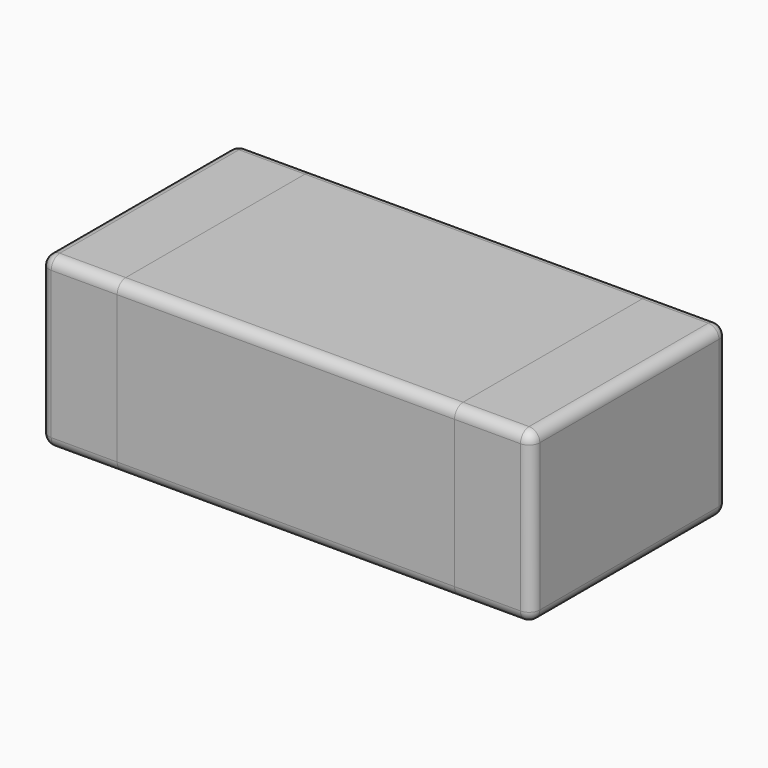
from build123d import *

# Parameters (mm, degrees)
F0_W           = 0.5
F0_H           = 1.6
F1_DEPTH       = 1.1
F0_W_2         = 2.2
F2_DEPTH       = 1.1
F3_R           = 0.07
F3_2_R         = 0.07
F4_T1_DEPTH    = 0.605
F4_S5_W        = 0.07
F4_S5_H        = 0.07
F4_T6_DEPTH    = 0.07
F4_S11_W       = 0.07
F4_S11_H       = 0.07
F4_T12_DEPTH   = 0.07
F4_S17_W       = 0.07
F4_S17_H       = 0.07
F4_T18_DEPTH   = 0.07
F4_S23_W       = 0.07
F4_S23_H       = 0.07
F4_T24_DEPTH   = 0.07
F4_2_F1_R      = 0.07
F4_2_F2_R      = 0.07
F4_2_F3_R      = 0.07
F4_2_F4_R      = 0.07
F4_3_T1_DEPTH  = 0.605
F4_3_S5_W      = 0.07
F4_3_S5_H      = 0.07
F4_3_T6_DEPTH  = 0.07
F4_3_S11_W     = 0.07
F4_3_S11_H     = 0.07
F4_3_T12_DEPTH = 0.07
F4_3_S17_W     = 0.07
F4_3_S17_H     = 0.07
F4_3_T18_DEPTH = 0.07
F4_3_S23_W     = 0.07
F4_3_S23_H     = 0.07
F4_3_T24_DEPTH = 0.07


# Not quite as in the source:
# - a fillet or chamfer that OpenCascade refuses, or shapes differently, is made with other operations: its cross-section is extruded or revolved along the edge and cut away or added


with BuildPart() as f1:
    # F0 (on Top) → F1 (new body)
    with BuildSketch(Plane.XY):
        with Locations((-1.35, 0)):
            Rectangle(F0_W, F0_H)
    extrude(amount=F1_DEPTH)

    # F3#2
    f3_2_edges = [f1.edges().sort_by_distance(p)[0] for p in [
        (-1.6, 0.8, 0.55),
        (-1.6, -0.8, 0.55),
        (-1.6, 0, 0),
        (-1.6, 0, 1.1),
    ]]
    fillet(f3_2_edges, radius=F3_2_R)

    # F4#3: fillet of radius 0.07 on 4 edges, made by hand

    # F4_3_s2 → F4_3_t1 (cut)
    with BuildSketch(Plane.YZ.offset(-1.53)):
        with BuildLine():
            ThreePointArc((0.73, 1.1), (0.7794974747, 1.0794974747), (0.8, 1.03))
            Line((0.8, 1.03), (0.8, 1.1))
            Line((0.8, 1.1), (0.73, 1.1))
        make_face()
        with BuildLine():
            ThreePointArc((0.73, 0), (0.7794974747, 0.0205025253), (0.8, 0.07))
            Line((0.8, 0.07), (0.8, 0))
            Line((0.8, 0), (0.73, 0))
        make_face()
        with BuildLine():
            ThreePointArc((-0.8, 1.03), (-0.7794974747, 1.0794974747), (-0.73, 1.1))
            Line((-0.73, 1.1), (-0.8, 1.1))
            Line((-0.8, 1.1), (-0.8, 1.03))
        make_face()
        with BuildLine():
            ThreePointArc((-0.8, 0.07), (-0.7794974747, 0.0205025253), (-0.73, 0))
            Line((-0.73, 0), (-0.8, 0))
            Line((-0.8, 0), (-0.8, 0.07))
        make_face()
    extrude(amount=F4_3_T1_DEPTH, mode=Mode.SUBTRACT)


with BuildPart() as f1b:
    # F0 (on Top) → F1, piece 2 (new body)
    with BuildSketch(Plane.XY):
        with Locations((1.35, 0)):
            Rectangle(F0_W, F0_H)
    extrude(amount=F1_DEPTH)

    # F3
    f3_edges = [f1b.edges().sort_by_distance(p)[0] for p in [
        (1.6, -0.8, 0.55),
        (1.6, 0.8, 0.55),
        (1.6, 0, 0),
        (1.6, 0, 1.1),
    ]]
    fillet(f3_edges, radius=F3_R)

    # F4: fillet of radius 0.07 on 4 edges, made by hand

    # F4_s2 → F4_t1 (cut)
    with BuildSketch(Plane.YZ.offset(0.925)):
        with BuildLine():
            ThreePointArc((0.73, 1.1), (0.7794974747, 1.0794974747), (0.8, 1.03))
            Line((0.8, 1.03), (0.8, 1.1))
            Line((0.8, 1.1), (0.73, 1.1))
        make_face()
        with BuildLine():
            ThreePointArc((0.73, 0), (0.7794974747, 0.0205025253), (0.8, 0.07))
            Line((0.8, 0.07), (0.8, 0))
            Line((0.8, 0), (0.73, 0))
        make_face()
        with BuildLine():
            ThreePointArc((-0.8, 1.03), (-0.7794974747, 1.0794974747), (-0.73, 1.1))
            Line((-0.73, 1.1), (-0.8, 1.1))
            Line((-0.8, 1.1), (-0.8, 1.03))
        make_face()
        with BuildLine():
            ThreePointArc((-0.8, 0.07), (-0.7794974747, 0.0205025253), (-0.73, 0))
            Line((-0.73, 0), (-0.8, 0))
            Line((-0.8, 0), (-0.8, 0.07))
        make_face()
    extrude(amount=F4_T1_DEPTH, mode=Mode.SUBTRACT)


with BuildPart() as f2:
    # F0 (on Top) → F2 (new body)
    with BuildSketch(Plane.XY):
        Rectangle(F0_W_2, F0_H)
    extrude(amount=F2_DEPTH)

    # F4#2: fillet of radius 0.07 on 4 edges, made by hand

    # F4_2_f1
    f4_2_f1_edges = [f2.edges().sort_by_distance(p)[0] for p in [
        (0, -0.8, 0),
    ]]
    fillet(f4_2_f1_edges, radius=F4_2_F1_R)

    # F4_2_f2
    f4_2_f2_edges = [f2.edges().sort_by_distance(p)[0] for p in [
        (0, -0.8, 1.1),
    ]]
    fillet(f4_2_f2_edges, radius=F4_2_F2_R)

    # F4_2_f3
    f4_2_f3_edges = [f2.edges().sort_by_distance(p)[0] for p in [
        (0, 0.8, 0),
    ]]
    fillet(f4_2_f3_edges, radius=F4_2_F3_R)

    # F4_2_f4
    f4_2_f4_edges = [f2.edges().sort_by_distance(p)[0] for p in [
        (0, 0.8, 1.1),
    ]]
    fillet(f4_2_f4_edges, radius=F4_2_F4_R)


with BuildPart() as f4_tool4:
    # F4_s5 → F4_t6 (new body)
    with BuildSketch(Plane.XZ.offset(0.73)):
        with Locations((1.565, 0.035)):
            Rectangle(F4_S5_W, F4_S5_H)
    extrude(amount=F4_T6_DEPTH)

    # F4_s7 → F4_t8 (revolve, cut)
    with BuildSketch(Plane(origin=(1.53, -0.73, 0.07), x_dir=(-0.7071067812, 0, 0.7071067812), z_dir=(0.7071067812, 0, 0.7071067812))):
        with BuildLine():
            ThreePointArc((0, -0.07), (0.07, 0), (0, 0.07))
            Line((0, 0.07), (0, -0.07))
        make_face()
    revolve(axis=Axis((1.53, -0.73, 0.07), (0, -1, 0)), mode=Mode.SUBTRACT)


with BuildPart() as f1b_1:
    add(f1b.part)

    # F4_t3: cut F4_tool4
    add(f4_tool4.part, mode=Mode.SUBTRACT)


with BuildPart() as f4_tool10:
    # F4_s11 → F4_t12 (new body)
    with BuildSketch(Plane.XZ.offset(0.73)):
        with Locations((1.565, 1.065)):
            Rectangle(F4_S11_W, F4_S11_H)
    extrude(amount=F4_T12_DEPTH)

    # F4_s13 → F4_t14 (revolve, cut)
    with BuildSketch(Plane(origin=(1.53, -0.73, 1.03), x_dir=(-0.7071067812, 0, -0.7071067812), z_dir=(-0.7071067812, 0, 0.7071067812))):
        with BuildLine():
            ThreePointArc((0, -0.07), (0.07, 0), (0, 0.07))
            Line((0, 0.07), (0, -0.07))
        make_face()
    revolve(axis=Axis((1.53, -0.73, 1.03), (0, -1, 0)), mode=Mode.SUBTRACT)


with BuildPart() as f1b_2:
    add(f1b_1.part)

    # F4_t9: cut F4_tool10
    add(f4_tool10.part, mode=Mode.SUBTRACT)


with BuildPart() as f4_tool16:
    # F4_s17 → F4_t18 (new body)
    with BuildSketch(Plane.XY.offset(0.07)):
        with Locations((1.565, 0.765)):
            Rectangle(F4_S17_W, F4_S17_H)
    extrude(amount=-F4_T18_DEPTH)

    # F4_s19 → F4_t20 (revolve, cut)
    with BuildSketch(Plane(origin=(1.53, 0.73, 0.07), x_dir=(-0.7071067812, -0.7071067812, 0), z_dir=(0.7071067812, -0.7071067812, 0))):
        with BuildLine():
            ThreePointArc((0, -0.07), (0.07, 0), (0, 0.07))
            Line((0, 0.07), (0, -0.07))
        make_face()
    revolve(axis=Axis((1.53, 0.73, 0.07), (0, 0, -1)), mode=Mode.SUBTRACT)


with BuildPart() as f1b_3:
    add(f1b_2.part)

    # F4_t15: cut F4_tool16
    add(f4_tool16.part, mode=Mode.SUBTRACT)


with BuildPart() as f4_tool22:
    # F4_s23 → F4_t24 (new body)
    with BuildSketch(Plane.XY.offset(1.03)):
        with Locations((1.565, 0.765)):
            Rectangle(F4_S23_W, F4_S23_H)
    extrude(amount=F4_T24_DEPTH)

    # F4_s25 → F4_t26 (revolve, cut)
    with BuildSketch(Plane(origin=(1.53, 0.73, 1.03), x_dir=(-0.7071067812, -0.7071067812, 0), z_dir=(-0.7071067812, 0.7071067812, 0))):
        with BuildLine():
            ThreePointArc((0, -0.07), (0.07, 0), (0, 0.07))
            Line((0, 0.07), (0, -0.07))
        make_face()
    revolve(axis=Axis((1.53, 0.73, 1.03), (0, 0, 1)), mode=Mode.SUBTRACT)


with BuildPart() as f1b_4:
    add(f1b_3.part)

    # F4_t21: cut F4_tool22
    add(f4_tool22.part, mode=Mode.SUBTRACT)


with BuildPart() as f4_3_tool4:
    # F4_3_s5 → F4_3_t6 (new body)
    with BuildSketch(Plane.XZ.offset(0.73)):
        with Locations((-1.565, 0.035)):
            Rectangle(F4_3_S5_W, F4_3_S5_H)
    extrude(amount=F4_3_T6_DEPTH)

    # F4_3_s7 → F4_3_t8 (revolve, cut)
    with BuildSketch(Plane(origin=(-1.53, -0.73, 0.07), x_dir=(0.7071067812, 0, 0.7071067812), z_dir=(0.7071067812, 0, -0.7071067812))):
        with BuildLine():
            ThreePointArc((0, -0.07), (0.07, 0), (0, 0.07))
            Line((0, 0.07), (0, -0.07))
        make_face()
    revolve(axis=Axis((-1.53, -0.73, 0.07), (0, -1, 0)), mode=Mode.SUBTRACT)


with BuildPart() as f1_1:
    add(f1.part)

    # F4_3_t3: cut F4_3_tool4
    add(f4_3_tool4.part, mode=Mode.SUBTRACT)


with BuildPart() as f4_3_tool10:
    # F4_3_s11 → F4_3_t12 (new body)
    with BuildSketch(Plane.XZ.offset(0.73)):
        with Locations((-1.565, 1.065)):
            Rectangle(F4_3_S11_W, F4_3_S11_H)
    extrude(amount=F4_3_T12_DEPTH)

    # F4_3_s13 → F4_3_t14 (revolve, cut)
    with BuildSketch(Plane(origin=(-1.53, -0.73, 1.03), x_dir=(0.7071067812, 0, -0.7071067812), z_dir=(-0.7071067812, 0, -0.7071067812))):
        with BuildLine():
            ThreePointArc((0, -0.07), (0.07, 0), (0, 0.07))
            Line((0, 0.07), (0, -0.07))
        make_face()
    revolve(axis=Axis((-1.53, -0.73, 1.03), (0, -1, 0)), mode=Mode.SUBTRACT)


with BuildPart() as f1_2:
    add(f1_1.part)

    # F4_3_t9: cut F4_3_tool10
    add(f4_3_tool10.part, mode=Mode.SUBTRACT)


with BuildPart() as f4_3_tool16:
    # F4_3_s17 → F4_3_t18 (new body)
    with BuildSketch(Plane.XY.offset(0.07)):
        with Locations((-1.565, 0.765)):
            Rectangle(F4_3_S17_W, F4_3_S17_H)
    extrude(amount=-F4_3_T18_DEPTH)

    # F4_3_s19 → F4_3_t20 (revolve, cut)
    with BuildSketch(Plane(origin=(-1.53, 0.73, 0.07), x_dir=(0.7071067812, -0.7071067812, 0), z_dir=(0.7071067812, 0.7071067812, 0))):
        with BuildLine():
            ThreePointArc((0, -0.07), (0.07, 0), (0, 0.07))
            Line((0, 0.07), (0, -0.07))
        make_face()
    revolve(axis=Axis((-1.53, 0.73, 0.07), (0, 0, -1)), mode=Mode.SUBTRACT)


with BuildPart() as f1_3:
    add(f1_2.part)

    # F4_3_t15: cut F4_3_tool16
    add(f4_3_tool16.part, mode=Mode.SUBTRACT)


with BuildPart() as f4_3_tool22:
    # F4_3_s23 → F4_3_t24 (new body)
    with BuildSketch(Plane.XY.offset(1.03)):
        with Locations((-1.565, 0.765)):
            Rectangle(F4_3_S23_W, F4_3_S23_H)
    extrude(amount=F4_3_T24_DEPTH)

    # F4_3_s25 → F4_3_t26 (revolve, cut)
    with BuildSketch(Plane(origin=(-1.53, 0.73, 1.03), x_dir=(0.7071067812, -0.7071067812, 0), z_dir=(-0.7071067812, -0.7071067812, 0))):
        with BuildLine():
            ThreePointArc((0, -0.07), (0.07, 0), (0, 0.07))
            Line((0, 0.07), (0, -0.07))
        make_face()
    revolve(axis=Axis((-1.53, 0.73, 1.03), (0, 0, 1)), mode=Mode.SUBTRACT)


with BuildPart() as f1_4:
    add(f1_3.part)

    # F4_3_t21: cut F4_3_tool22
    add(f4_3_tool22.part, mode=Mode.SUBTRACT)


solid = Compound([f2.part, f1b_4.part, f1_4.part])
